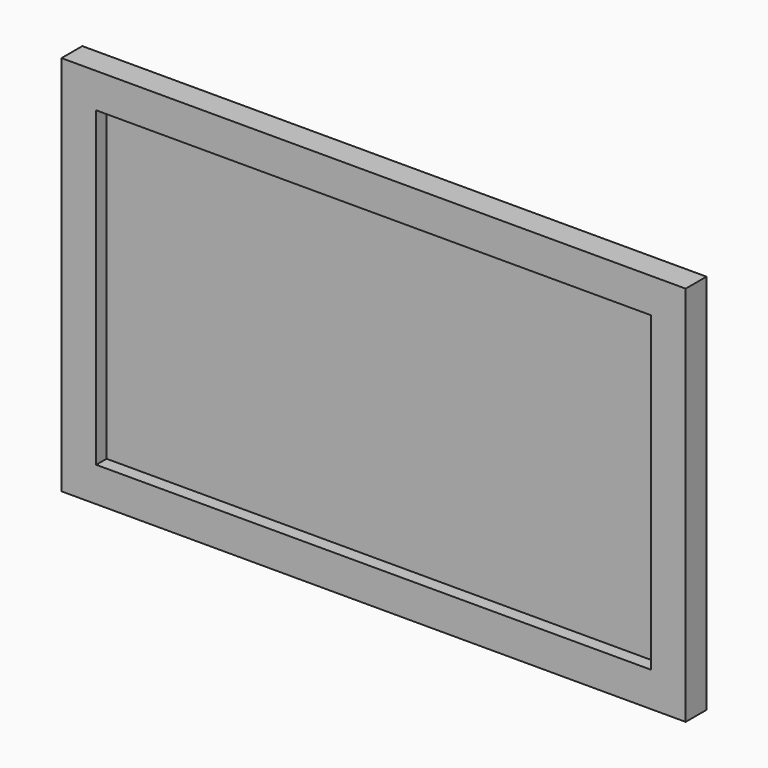
from build123d import *

# Parameters (mm, degrees)
F0_W        = 406.4
F0_H        = 228.6
F1_DEPTH    = 12.7
F2_W        = 457.2
F2_H        = 279.4
F2_W_2      = 406.4
F2_H_2      = 228.6
F3_DEPTH    = 9.525
F4_W        = 419.1
F4_H        = 241.3
F5_DEPTH    = 25.4
F6_T1_DEPTH = 525.2806331425
F6_T3_DEPTH = 703.0806331425


# Not quite as in the source:
# - a fillet or chamfer that OpenCascade refuses, or shapes differently, is made with other operations: its cross-section is extruded or revolved along the edge and cut away or added


with BuildPart() as f1:
    # F0 (on Front) → F1 (new body)
    with BuildSketch(Plane.XZ):
        Rectangle(F0_W, F0_H)
    extrude(amount=F1_DEPTH)


with BuildPart() as f3:
    # F2 (on face) → F3 (new body, symmetric)
    with BuildSketch(Plane.XZ.offset(12.7)):
        Rectangle(F2_W, F2_H)
        Rectangle(F2_W_2, F2_H_2, mode=Mode.SUBTRACT)
    extrude(amount=F3_DEPTH, both=True)

    # F4 (on face) → F5 (join)
    with BuildSketch(Plane(origin=(0, -3.175, 0), x_dir=(-1, 0, 0), z_dir=(0, 1, 0))):
        Rectangle(F4_W, F4_H)
    extrude(amount=F5_DEPTH)

    # F6: fillet of radius 76.2 on 4 edges, made by hand

    # F6_s2 → F6_t1 (cut)
    with BuildSketch(Plane.XY.offset(-262.6403165712)):
        with BuildLine():
            ThreePointArc((209.55, -3.175), (183.8623931049, 15.5857648032), (152.7538733715, 22.225))
            Line((152.7538733715, 22.225), (209.55, 22.225))
            Line((209.55, 22.225), (209.55, -3.175))
        make_face()
        with BuildLine():
            ThreePointArc((-209.55, -3.175), (-183.8623931049, 15.5857648032), (-152.7538733715, 22.225))
            Line((-152.7538733715, 22.225), (-209.55, 22.225))
            Line((-209.55, 22.225), (-209.55, -3.175))
        make_face()
    extrude(amount=F6_T1_DEPTH, mode=Mode.SUBTRACT)

    # F6_s4 → F6_t3 (cut)
    with BuildSketch(Plane.YZ.offset(-351.5403165712)):
        with BuildLine():
            ThreePointArc((-3.175, 120.65), (15.5857648032, 94.9623931049), (22.225, 63.8538733715))
            Line((22.225, 63.8538733715), (22.225, 120.65))
            Line((22.225, 120.65), (-3.175, 120.65))
        make_face()
        with BuildLine():
            ThreePointArc((-3.175, -120.65), (15.5857648032, -94.9623931049), (22.225, -63.8538733715))
            Line((22.225, -63.8538733715), (22.225, -120.65))
            Line((22.225, -120.65), (-3.175, -120.65))
        make_face()
    extrude(amount=F6_T3_DEPTH, mode=Mode.SUBTRACT)


solid = Compound([f1.part, f3.part])
